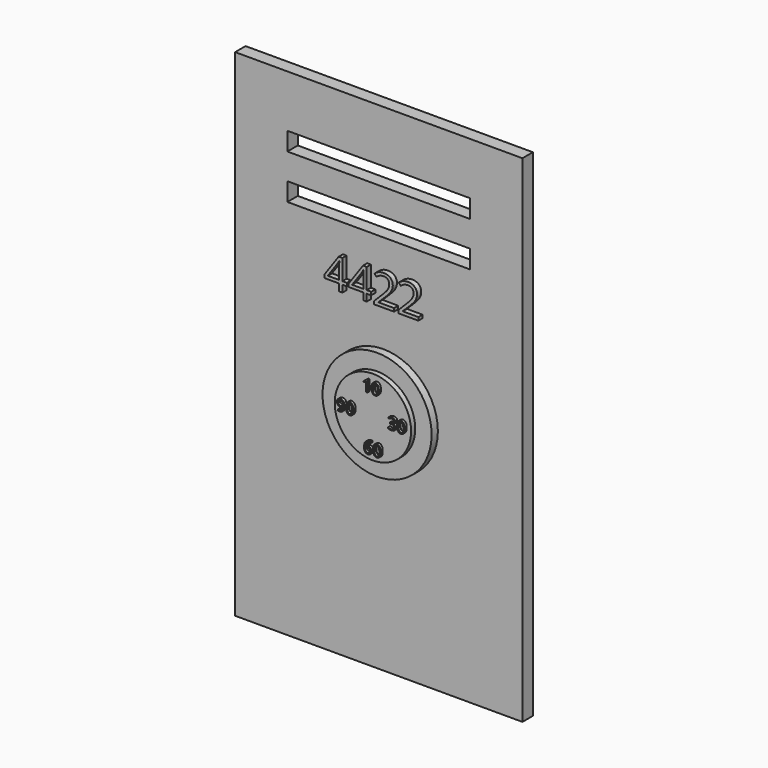
from build123d import *

# Parameters (mm, degrees)
F0_W            = 279.4
F0_H            = 482.6
F1_DEPTH        = 12.7
F2_W            = 177.8
F2_H            = 17.78
F3_DEPTH        = 25.4
F4_TEXT_SIZE    = 41.3300469518
F5_DEPTH        = 5.08
F6_R            = 53.0421933998
F7_DEPTH        = 7.62
F8_R            = 37.1245625736
F9_DEPTH        = 12.7
F10_TEXT_SIZE   = 15.5959045514
F10_TEXT_SIZE_2 = 15.3270084411
F10_TEXT_SIZE_3 = 15.3270032671
F10_TEXT_SIZE_4 = 15.0581097437
F11_DEPTH       = 2.54


# Not quite as in the source:
# - Text() gives the source's letters only with a copy of the font that has no kerning and outlines rounded to 1/6400 em; it was checked with that copy


with BuildPart() as f1:
    # F0 (on Front) → F1 (new body)
    with BuildSketch(Plane.XZ):
        with Locations((-4.4300854206, 68.9326664422)):
            Rectangle(F0_W, F0_H)
    extrude(amount=F1_DEPTH)

    # F2 (on face) → F3 (cut)
    with BuildSketch(Plane.XZ.offset(12.7)):
        with Locations((-4.4300854206, 250.5426664422)):
            Rectangle(F2_W, F2_H)
        with Locations((-4.4300854206, 207.3626664422)):
            Rectangle(F2_W, F2_H)
    extrude(amount=-F3_DEPTH, mode=Mode.SUBTRACT)

    # F4 (on face) → F5 (join)
    with BuildSketch(Plane.XZ.offset(12.7)):
        with Locations((-54.1678434238, 141.6262984276)):
            Text('4422', F4_TEXT_SIZE, font='Open Sans', text_align=(TextAlign.LEFT, TextAlign.BOTTOM))
    extrude(amount=F5_DEPTH)

    # F6 (on face) → F7 (join)
    with BuildSketch(Plane.XZ.offset(12.7)):
        with Locations((0, 49.8027577996)):
            Circle(F6_R)
    extrude(amount=F7_DEPTH)

    # F8 (on face) → F9 (join)
    with BuildSketch(Plane.XZ.offset(12.7)):
        with Locations((0, 49.8027577996)):
            Circle(F8_R)
    extrude(amount=F9_DEPTH)

    # F10 (on face) → F11 (join)
    with BuildSketch(Plane.XZ.offset(25.4)):
        with Locations((-7.493824698, 18.1903652847)):
            Text('60', F10_TEXT_SIZE, font='Open Sans', text_align=(TextAlign.LEFT, TextAlign.BOTTOM))
        with Locations((-33.6304008961, 45.8757765591)):
            Text('90', F10_TEXT_SIZE_2, font='Open Sans', text_align=(TextAlign.LEFT, TextAlign.BOTTOM))
        with Locations((16.125895083, 46.0693836212)):
            Text('30', F10_TEXT_SIZE_3, font='Open Sans', text_align=(TextAlign.LEFT, TextAlign.BOTTOM))
        with Locations((-8.6554503068, 70.6571266055)):
            Text('10', F10_TEXT_SIZE_4, font='Open Sans', text_align=(TextAlign.LEFT, TextAlign.BOTTOM))
    extrude(amount=F11_DEPTH)


solid = f1.part
